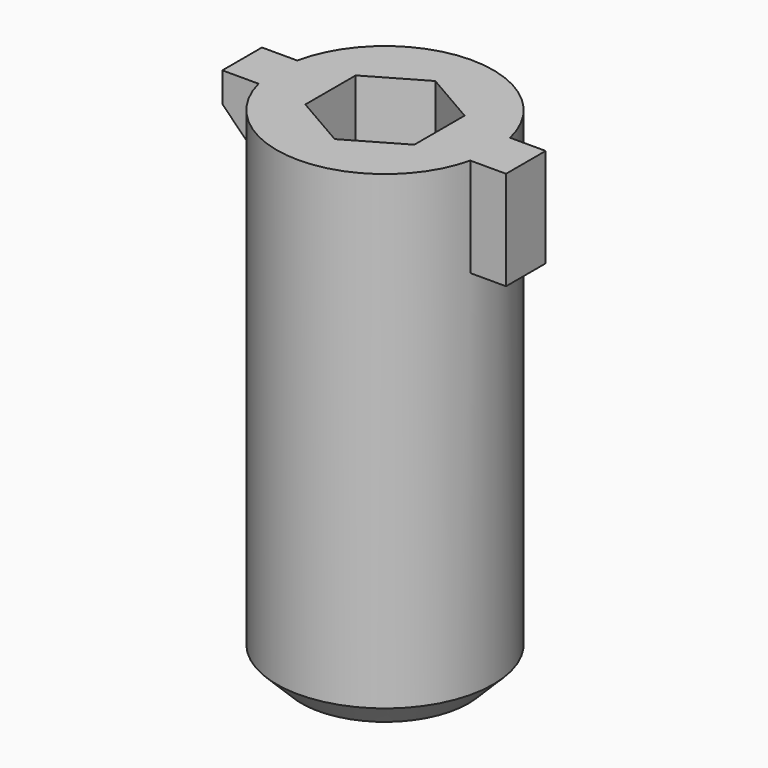
from build123d import *

# Parameters (mm, degrees)
F0_R        = 4.375
F1_DEPTH    = 20
F2_W        = 2
F2_H        = 4
F3_DEPTH    = 3.5
F4_W        = 2
F4_H        = 4
F5_DEPTH    = 3.5
F6_T4_DEPTH = 16.4014247326
F6_S5_R     = 4.375
F6_T6_DEPTH = 10
F7_SIZE     = 1
F8_SIZE     = 0.4


# Not quite as in the source:
# - a fillet or chamfer that OpenCascade refuses, or shapes differently, is made with other operations: its cross-section is extruded or revolved along the edge and cut away or added


with BuildPart() as f1:
    # F0 (on Top) → F1 (new body)
    with BuildSketch(Plane.XY):
        Circle(F0_R)
        Polygon((-2.2, -1.2701705922), (-2.2, 1.2701705922), (0, 2.5403411844), (2.2, 1.2701705922), (2.2, -1.2701705922), (0, -2.5403411844), align=None, mode=Mode.SUBTRACT)
    extrude(amount=F1_DEPTH)

    # F2 (on face) → F3 (join)
    with BuildSketch(Plane.YZ.offset(-2.2)):
        with Locations((-0.0866705922, 18)):
            Rectangle(F2_W, F2_H)
    extrude(amount=-F3_DEPTH)

    # F4 (on face) → F5 (join)
    with BuildSketch(Plane(origin=(2.2, 0, 0), x_dir=(0, -1, 0), z_dir=(-1, 0, 0))):
        with Locations((0.0136538511, 18)):
            Rectangle(F4_W, F4_H)
    extrude(amount=-F5_DEPTH)

    # F6: chamfer of 2.8 on 1 edges, made by hand


with BuildPart() as f6_tool2:
    # F6_s3 → F6_t4 (new body)
    with BuildSketch(Plane.XZ.offset(8.2873829585)):
        Polygon((-5.7, 18.8), (-2.9, 16), (-5.7, 16), align=None)
    extrude(amount=-F6_T4_DEPTH)

    # F6_s5 → F6_t6 (cut, symmetric)
    with BuildSketch(Plane.XY.offset(17.4)):
        Circle(F6_S5_R)
    extrude(amount=F6_T6_DEPTH, both=True, mode=Mode.SUBTRACT)


with BuildPart() as f1_1:
    add(f1.part)

    # F6_t1: cut F6_tool2
    add(f6_tool2.part, mode=Mode.SUBTRACT)

    # F7
    f7_edges = [f1_1.edges().sort_by_distance(p)[0] for p in [
        (-4.375, 0, 0),
    ]]
    chamfer(f7_edges, length=F7_SIZE)

    # F8
    f8_edges = [f1_1.edges().sort_by_distance(p)[0] for p in [
        (2.2, 0, 0),
        (1.1, -1.905256, 0),
        (-1.1, -1.905256, 0),
        (-2.2, 0, 0),
        (-1.1, 1.905256, 0),
        (1.1, 1.905256, 0),
    ]]
    chamfer(f8_edges, length=F8_SIZE)


solid = f1_1.part
